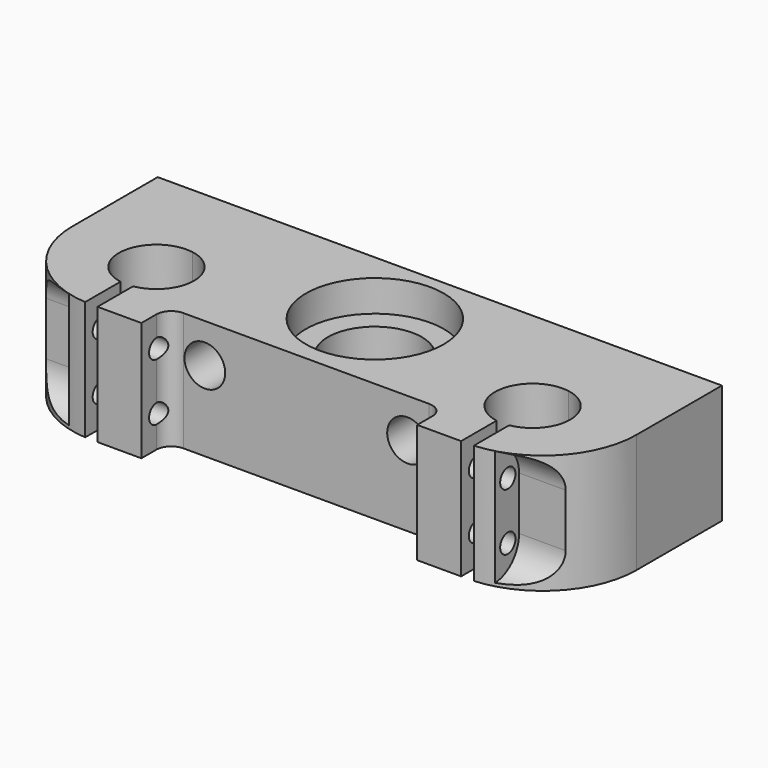
from build123d import *

# Parameters (mm, degrees)
F0_R      = 11
F1_DEPTH  = 25
F3_R      = 1.525
F4_DEPTH  = 105.2
F5_DEPTH  = 11
F7_DEPTH  = 11
F0_R_2    = 7.5
F8_DEPTH  = 20
F9_DEPTH  = 5
F10_R     = 2
F11_DEPTH = 10
F13_DEPTH = 25.0010001
F14_DEPTH = 6
F15_DEPTH = 10
F16_R     = 3.25
F17_DEPTH = 25


# Not quite as in the source:
# - a feature names something its author has since deleted; it is built from what else it names


with BuildPart() as f1:
    # F0 (on Top) → F1 (new body)
    with BuildSketch(Plane.XY):
        with BuildLine():
            Line((90, -8), (0, -8))
            Line((0, -8), (0, -25))
            ThreePointArc((0, -25), (4.0455488499, -35.246950766), (14, -39.9666295471))
            Line((14, -39.9666295471), (14, -32.9160797831))
            ThreePointArc((14, -32.9160797831), (9, -27), (14, -21.0839202169))
            Line((14, -21.0839202169), (14, -14))
            Line((14, -14), (16, -14))
            Line((16, -14), (16, -21.0839202169))
            ThreePointArc((16, -21.0839202169), (19.582575695, -23.1270166538), (21, -27))
            ThreePointArc((21, -27), (19.582575695, -30.8729833462), (16, -32.9160797831))
            Line((16, -32.9160797831), (16, -40))
            Line((16, -40), (74, -40))
            Line((74, -40), (74, -32.9160797831))
            ThreePointArc((74, -32.9160797831), (69, -27), (74, -21.0839202169))
            Line((74, -21.0839202169), (74, -14))
            Line((74, -14), (76, -14))
            Line((76, -14), (76, -21.0839202169))
            ThreePointArc((76, -21.0839202169), (79.582575695, -23.1270166538), (81, -27))
            ThreePointArc((81, -27), (79.582575695, -30.8729833462), (76, -32.9160797831))
            Line((76, -32.9160797831), (76, -39.9666295471))
            ThreePointArc((76, -39.9666295471), (85.9544511501, -35.246950766), (90, -25))
            Line((90, -25), (90, -8))
        make_face()
        with Locations((45, -20.9553470761)):
            Circle(F0_R, mode=Mode.SUBTRACT)
        with BuildLine():
            Line((14, -14), (14, -21.0839202169))
            ThreePointArc((14, -21.0839202169), (15, -21), (16, -21.0839202169))
            Line((16, -21.0839202169), (16, -14))
            Line((16, -14), (14, -14))
        make_face()
        with BuildLine():
            ThreePointArc((74, -21.0839202169), (75, -21), (76, -21.0839202169))
            Line((76, -21.0839202169), (76, -14))
            Line((76, -14), (74, -14))
            Line((74, -14), (74, -21.0839202169))
        make_face()
    extrude(amount=F1_DEPTH)

    # F3 (on Right) → F4 (cut)
    with BuildSketch(Plane.YZ):
        with Locations((-36.9413755834, 11.0567829106)):
            Circle(F3_R)
        with Locations((-36.9413755834, 20.1872170437)):
            Circle(F3_R)
    extrude(amount=F4_DEPTH, mode=Mode.SUBTRACT)

    # F3 (on Right) → F5 (cut)
    with BuildSketch(Plane.YZ):
        with BuildLine():
            Line((-39.7998355329, 24.9966811389), (-39.7998355329, 6.4961747266))
            Line((-39.7998355329, 6.4961747266), (-39.6976853907, 6.4961747266))
            ThreePointArc((-39.6976853907, 6.4961747266), (-36.1621514848, 7.9606408207), (-34.6976853907, 11.4961747266))
            Line((-34.6976853907, 11.4961747266), (-34.6976853907, 19.9966811389))
            ThreePointArc((-34.6976853907, 19.9966811389), (-36.1621514848, 23.5322150448), (-39.6976853907, 24.9966811389))
            Line((-39.6976853907, 24.9966811389), (-39.7998355329, 24.9966811389))
        make_face()
        with Locations((-36.9413755834, 11.0567829106)):
            Circle(F3_R, mode=Mode.SUBTRACT)
        with Locations((-36.9413755834, 20.1872170437)):
            Circle(F3_R, mode=Mode.SUBTRACT)
    extrude(amount=F5_DEPTH, mode=Mode.SUBTRACT)

    # F6 (on offset) → F7 (cut)
    with BuildSketch(Plane.YZ.offset(90)):
        with BuildLine():
            Line((-39.7998355329, 24.9966811389), (-39.7998355329, 6.4961747266))
            Line((-39.7998355329, 6.4961747266), (-39.6976853907, 6.4961747266))
            ThreePointArc((-39.6976853907, 6.4961747266), (-36.1621514848, 7.9606408207), (-34.6976853907, 11.4961747266))
            Line((-34.6976853907, 11.4961747266), (-34.6976853907, 19.9966811389))
            ThreePointArc((-34.6976853907, 19.9966811389), (-36.1621514848, 23.5322150448), (-39.6976853907, 24.9966811389))
            Line((-39.6976853907, 24.9966811389), (-39.7998355329, 24.9966811389))
        make_face()
    extrude(amount=-F7_DEPTH, mode=Mode.SUBTRACT)

    # F0 (on Top) → F8 (join)
    with BuildSketch(Plane.XY):
        with Locations((45, -20.9553470761)):
            Circle(F0_R)
        with Locations((45, -20.9553470761)):
            Circle(F0_R_2, mode=Mode.SUBTRACT)
    extrude(amount=F8_DEPTH)

    # F0 (on Top) → F9 (cut)
    with BuildSketch(Plane.XY):
        with Locations((45, -20.9553470761)):
            Circle(F0_R)
        with Locations((45, -20.9553470761)):
            Circle(F0_R_2, mode=Mode.SUBTRACT)
    extrude(amount=F9_DEPTH, mode=Mode.SUBTRACT)

    # F10 (on face) → F11 (cut)
    with BuildSketch(Plane(origin=(0, -8, 0), x_dir=(-1, 0, 0), z_dir=(0, 1, 0))):
        with Locations((-28.83, 18.75)):
            Circle(F10_R)
        with Locations((-61.17, 18.75)):
            Circle(F10_R)
    extrude(amount=-F11_DEPTH, mode=Mode.SUBTRACT)

    # F12 (on face) → F13 (cut, through all)
    with BuildSketch(Plane.XY.offset(25)):
        with BuildLine():
            Line((45, -40), (45, -34.6395410597))
            Line((45, -34.6395410597), (25.387, -34.6395410597))
            ThreePointArc((25.387, -34.6395410597), (23.6991374304, -35.338675856), (23, -37.0265373344))
            Line((23, -37.0265373344), (23, -40))
            Line((23, -40), (45, -40))
        make_face()
        with BuildLine():
            ThreePointArc((67, -36.7889047916), (66.2265029782, -35.2566531011), (64.6248583192, -34.6395410597))
            Line((64.6248583192, -34.6395410597), (45, -34.6395410597))
            Line((45, -34.6395410597), (45, -40))
            Line((45, -40), (67, -40))
            Line((67, -40), (67, -36.7889047916))
        make_face()
    extrude(amount=-F13_DEPTH, mode=Mode.SUBTRACT)

    # F0 (on Top) → F14 (cut)
    with BuildSketch(Plane.XY):
        with BuildLine():
            Line((90, -8), (0, -8))
            Line((0, -8), (0, -25))
            ThreePointArc((0, -25), (4.0455488499, -35.246950766), (14, -39.9666295471))
            Line((14, -39.9666295471), (14, -32.9160797831))
            ThreePointArc((14, -32.9160797831), (9, -27), (14, -21.0839202169))
            Line((14, -21.0839202169), (14, -14))
            Line((14, -14), (16, -14))
            Line((16, -14), (16, -21.0839202169))
            ThreePointArc((16, -21.0839202169), (19.582575695, -23.1270166538), (21, -27))
            ThreePointArc((21, -27), (19.582575695, -30.8729833462), (16, -32.9160797831))
            Line((16, -32.9160797831), (16, -40))
            Line((16, -40), (74, -40))
            Line((74, -40), (74, -32.9160797831))
            ThreePointArc((74, -32.9160797831), (69, -27), (74, -21.0839202169))
            Line((74, -21.0839202169), (74, -14))
            Line((74, -14), (76, -14))
            Line((76, -14), (76, -21.0839202169))
            ThreePointArc((76, -21.0839202169), (79.582575695, -23.1270166538), (81, -27))
            ThreePointArc((81, -27), (79.582575695, -30.8729833462), (76, -32.9160797831))
            Line((76, -32.9160797831), (76, -39.9666295471))
            ThreePointArc((76, -39.9666295471), (85.9544511501, -35.246950766), (90, -25))
            Line((90, -25), (90, -8))
        make_face()
        with Locations((45, -20.9553470761)):
            Circle(F0_R, mode=Mode.SUBTRACT)
        with BuildLine():
            Line((14, -14), (14, -21.0839202169))
            ThreePointArc((14, -21.0839202169), (15, -21), (16, -21.0839202169))
            Line((16, -21.0839202169), (16, -14))
            Line((16, -14), (14, -14))
        make_face()
        with BuildLine():
            ThreePointArc((74, -21.0839202169), (75, -21), (76, -21.0839202169))
            Line((76, -21.0839202169), (76, -14))
            Line((76, -14), (74, -14))
            Line((74, -14), (74, -21.0839202169))
        make_face()
        with Locations((45, -20.9553470761)):
            Circle(F0_R)
        with Locations((45, -20.9553470761)):
            Circle(F0_R_2, mode=Mode.SUBTRACT)
    extrude(amount=F14_DEPTH, mode=Mode.SUBTRACT)

    # F0 (on Top) → F15 (cut)
    with BuildSketch(Plane.XY):
        with Locations((45, -20.9553470761)):
            Circle(F0_R)
        with Locations((45, -20.9553470761)):
            Circle(F0_R_2, mode=Mode.SUBTRACT)
    extrude(amount=F15_DEPTH, mode=Mode.SUBTRACT)

    # F16 (on face) → F17 (cut)
    with BuildSketch(Plane.XZ.offset(40)):
        with Locations((28.83, 18.75)):
            Circle(F16_R)
        with Locations((61.17, 18.75)):
            Circle(F16_R)
    extrude(amount=-F17_DEPTH, mode=Mode.SUBTRACT)


solid = f1.part
